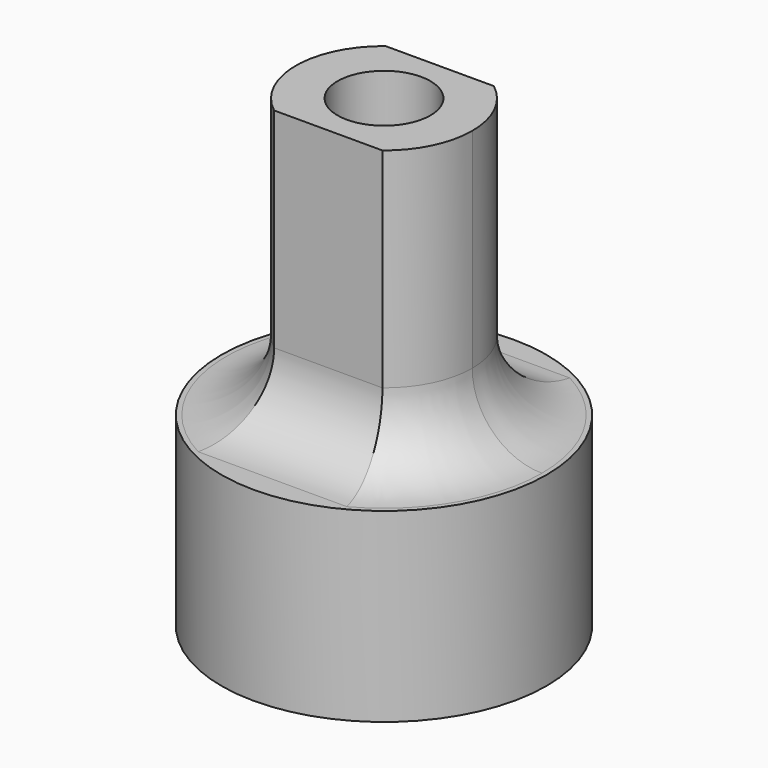
from build123d import *

# Parameters (mm, degrees)
F0_W     = 2.3323807579
F0_H     = 3
F1_DEPTH = 10
F2_R     = 3.5
F3_DEPTH = 4
F4_R     = 1.5
F5_R     = 1
F6_DEPTH = 25


with BuildPart() as f1:
    # F0 (on Top) → F1 (new body)
    with BuildSketch(Plane.XY):
        with BuildLine():
            Line((-1.166190379, -1.5), (-1.166190379, 1.5))
            ThreePointArc((-1.166190379, 1.5), (-1.9, 0), (-1.166190379, -1.5))
        make_face()
        with BuildLine():
            ThreePointArc((1.166190379, -1.5), (1.7067163971, -0.8349366084), (1.9, 0))
            ThreePointArc((1.9, 0), (1.7067163971, 0.8349366084), (1.166190379, 1.5))
            Line((1.166190379, 1.5), (1.166190379, -1.5))
        make_face()
        Rectangle(F0_W, F0_H)
    extrude(amount=F1_DEPTH)

    # F2 (on Top) → F3 (join)
    with BuildSketch(Plane.XY):
        Circle(F2_R)
    extrude(amount=F3_DEPTH)

    # F4
    f4_edges = [f1.edges().sort_by_distance(p)[0] for p in [
        (-1.9, 0, 4),
        (0, 1.5, 4),
        (0, -1.5, 4),
        (1.9, 0, 4),
    ]]
    fillet(f4_edges, radius=F4_R)

    # F5 (on face) → F6 (cut)
    with BuildSketch(Plane.XY.offset(10)):
        Circle(F5_R)
    extrude(amount=-F6_DEPTH, mode=Mode.SUBTRACT)


solid = f1.part
